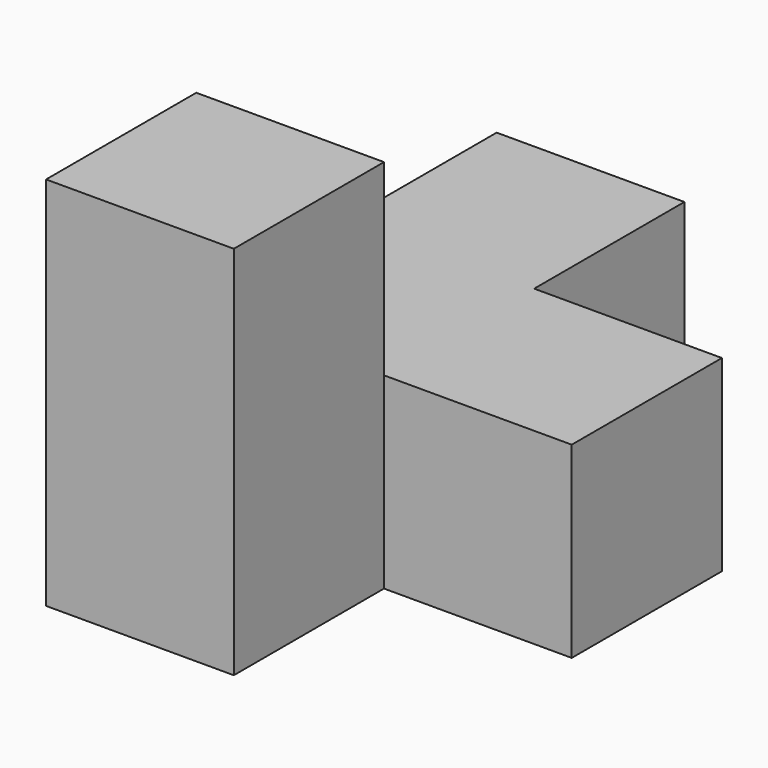
from build123d import *

# Parameters (mm, degrees)
F1_W     = 127
F1_H     = 127
F2_DEPTH = 190.5
F3_W     = 127
F3_H     = 127
F4_DEPTH = 127
F5_W     = 127
F5_H     = 127
F6_DEPTH = 127


# Not quite as in the source:
# - a variable given as a bare number and used for a length is read in inches; the dataset says mm whatever the document's units were


with BuildPart() as f2:
    # F1 (on Front) → F2 (new body, symmetric)
    with BuildSketch(Plane.XZ):
        Rectangle(F1_W, F1_H)
    extrude(amount=F2_DEPTH, both=True)

    # F3 (on face) → F4 (join)
    with BuildSketch(Plane.XY.offset(63.5)):
        with Locations((0, -127)):
            Rectangle(F3_W, F3_H)
    extrude(amount=F4_DEPTH)

    # F5 (on face) → F6 (join)
    with BuildSketch(Plane.YZ.offset(63.5)):
        Rectangle(F5_W, F5_H)
    extrude(amount=F6_DEPTH)


solid = f2.part
